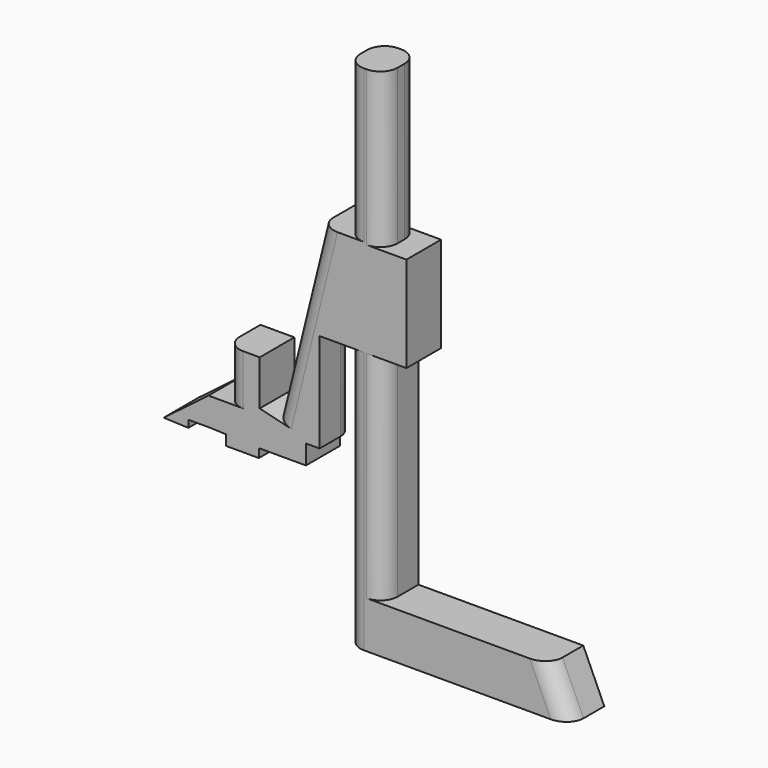
from build123d import *

# Parameters (mm, degrees)
F0_W     = 7.8990748152
F0_H     = 28.538595885
F0_W_2   = 6.6250311211
F0_H_2   = 28.0289780349
F1_DEPTH = 12.7
F2_R     = 5.08


# Not quite as in the source:
# - two fillets or chamfers of one size are made in one step


with BuildPart() as f1:
    # F0 (on Front) → F1 (new body)
    with BuildSketch(Plane.XZ):
        Polygon((10.9567856416, 73.384962976), (0, 73.384962976), (0, 28.538595885), (0, 0), (0, -76.9523009658), (10.9567856416, -76.9523009658), (10.9567856416, -63.2497891784), (10.9567856416, -57.5868189335), (10.9567856416, 0), (10.9567856416, 28.0289780349), align=None)
        with Locations((-3.9495374076, 14.2692979425)):
            Rectangle(F0_W, F0_H)
        with Locations((14.2693012021, 14.0144890174)):
            Rectangle(F0_W_2, F0_H_2)
        Polygon((-7.8990748152, 0), (-7.8990748152, 28.538595885), (-21.1491379887, -25.4808943719), (-25.4754136512, -24.4197324549), (-25.7356986403, -29.0482211858), (-11.9106527418, -29.0482211858), (-7.8990748152, -29.0482211858), align=None)
        Polygon((10.9567856416, -63.2497891784), (10.9567856416, -76.9523009658), (65.48589468, -76.9523009658), (59.3128465116, -63.2497891784), align=None)
        Polygon((-25.7356986403, -29.0482211858), (-25.4754136512, -24.4197324549), (-25.4754136512, -11.2115936354), (-35.4184396565, -11.2115936354), (-35.4184396565, -25.9905140847), (-40.5146181583, -25.9905140847), (-53.649477917, -35.9711753499), (-46.4077852666, -36.2483747303), (-46.4077852666, -34.144397825), (-40.0049984455, -34.144397825), (-35.4184396565, -34.3199633062), (-35.4184396565, -37.3197160661), (-25.7356986403, -37.3197160661), (-25.7356986403, -34.7485020757), (-11.9106527418, -34.7485020757), (-11.9106527418, -29.0482211858), align=None)
    extrude(amount=F1_DEPTH)

    # F2
    f2_edges = [f1.edges().sort_by_distance(p)[0] for p in [
        (-35.41844, -12.7, -18.601054),
        (10.956786, -12.7, -31.624895),
        (0, -12.7, 50.961779),
        (0, -12.7, -38.47615),
        (0, 0, 50.961779),
        (-14.524106, -12.7, 1.528851),
        (-7.899075, 0, -14.524111),
        (62.399371, -12.7, -70.101045),
        (10.956786, 0, 50.706971),
        (10.956786, -12.7, 50.706971),
    ]]
    fillet(f2_edges, radius=F2_R)


solid = f1.part
